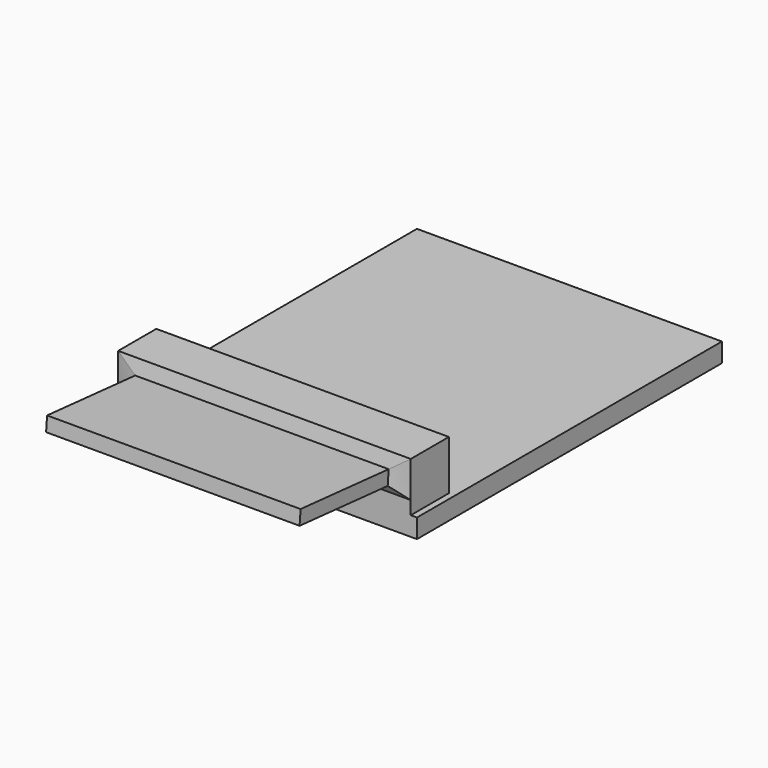
from build123d import *

# Parameters (mm, degrees)
F0_W      = 16
F0_H      = 20
F1_DEPTH  = 1
F2_W      = 15.35
F2_H      = 2.5
F3_DEPTH  = 2.6
F7_W      = 13.3
F7_H      = 0.75
F8_DEPTH  = 5.8
F4_W      = 15.35
F4_H      = 1.9
F8_FACE_W = 13.3
F8_FACE_H = 0.75


with BuildPart() as f1:
    # F0 (on Top) → F1 (new body)
    with BuildSketch(Plane.XY):
        Rectangle(F0_W, F0_H)
    extrude(amount=F1_DEPTH)

    # F2 (on face) → F3 (join)
    with BuildSketch(Plane.XY.offset(1)):
        with Locations((0, -8.75)):
            Rectangle(F2_W, F2_H)
    extrude(amount=F3_DEPTH)



with BuildPart() as f8:
    # F7 (on face) → F8 (new body)
    with BuildSketch(Plane(origin=(0, -10.3362249547, 0.9043025072), x_dir=(-1, 0, 0), z_dir=(0, 0.9961946981, -0.0871557427))):
        with Locations((0, 1.5897434857)):
            Rectangle(F7_W, F7_H)
    extrude(amount=-F8_DEPTH)


with BuildPart() as f1_1:
    add(f1.part)

    add(f8.part)  # F9 merges F8
    # F4 (on face) → F9 section 0
    with BuildSketch(Plane.XZ.offset(10)):
        with Locations((0, 2.65)):
            Rectangle(F4_W, F4_H)
    # F8_face (on face) → F9 section 1
    with BuildSketch(Plane(origin=(0, -10.1976696804, 2.4879965389), x_dir=(-1, 0, 0), z_dir=(0, 0.9961946981, -0.0871557427))):
        Rectangle(F8_FACE_W, F8_FACE_H)
    loft()


solid = f1_1.part
